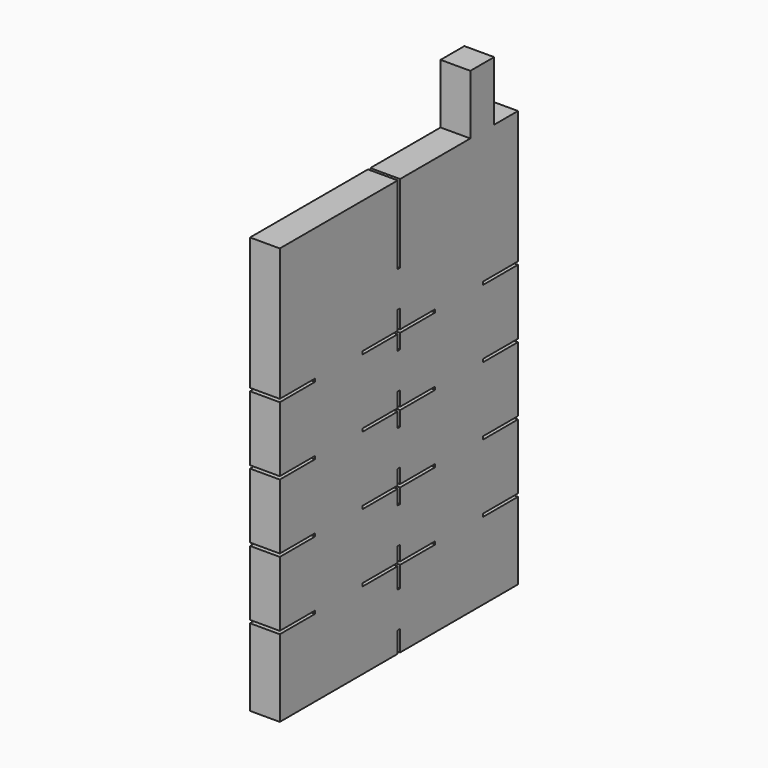
from build123d import *

# Parameters (mm, degrees)
F1_DEPTH = 5
F2_DEPTH = 10


# Not quite as in the source:
# - a feature names something its author has since deleted; it is built from what else it names


with BuildPart() as f1:
    # F0 (on Right) → F1 (new body)
    with BuildSketch(Plane.YZ):
        Polygon((11.5, 0), (0, 0), (0, -12.238), (7.3750000447, -12.238), (7.3750000447, -12.738), (0, -12.738), (0, -23.672), (7.3750000447, -23.672), (7.3750000447, -24.172), (0, -24.172), (0, -35.106), (7.3750000447, -35.106), (7.3750000447, -35.606), (0, -35.606), (0, -46.54), (7.3750000447, -46.54), (7.3750000447, -47.04), (0, -47.04), (0, -60), (24.75, -60), (24.75, -56.52), (25.25, -56.52), (25.25, -60), (50, -60), (50, -47.04), (42.6249988377, -47.04), (42.6249988377, -46.54), (50, -46.54), (50, -35.606), (42.6249988377, -35.606), (42.6249988377, -35.106), (50, -35.106), (50, -24.172), (42.6249988377, -24.172), (42.6249988377, -23.672), (50, -23.672), (50, -12.738), (42.6249988377, -12.738), (42.6249988377, -12.238), (50, -12.238), (50, 0), (45, 0), (45, 15), (45, 19.999999553), (40, 19.999999553), (40, 15), (40, 0), (37.625, 0), (35.125, 0), (25.25, 0), (25.25, -1.304), (25.25, -3.119), (24.75, -3.119), (24.75, 0), (14.875, 0), (12.375, 0), align=None)
        Polygon((25.25, -44.073), (25.25, -46.54), (32.625, -46.54), (32.625, -47.04), (25.25, -47.04), (25.25, -50.52), (24.75, -50.52), (24.75, -47.04), (17.375, -47.04), (17.375, -46.54), (24.75, -46.54), (24.75, -44.073), align=None, mode=Mode.SUBTRACT)
        Polygon((25.25, -32.639), (25.25, -35.106), (32.625, -35.106), (32.625, -35.606), (25.25, -35.606), (25.25, -38.073), (24.75, -38.073), (24.75, -35.606), (17.375, -35.606), (17.375, -35.106), (24.75, -35.106), (24.75, -32.639), align=None, mode=Mode.SUBTRACT)
        Polygon((25.25, -21.205), (25.25, -23.672), (32.625, -23.672), (32.625, -24.172), (25.25, -24.172), (25.25, -26.639), (24.75, -26.639), (24.75, -24.172), (17.375, -24.172), (17.375, -23.672), (24.75, -23.672), (24.75, -21.205), align=None, mode=Mode.SUBTRACT)
        Polygon((25.25, -9.119), (25.25, -12.238), (32.625, -12.238), (32.625, -12.738), (25.25, -12.738), (25.25, -15.205), (24.75, -15.205), (24.75, -12.738), (17.375, -12.738), (17.375, -12.238), (24.75, -12.238), (24.75, -9.119), align=None, mode=Mode.SUBTRACT)
    extrude(amount=F1_DEPTH)

    # F2 (add): faces of the model
    f2_faces = [f1.faces().sort_by_distance(p)[0] for p in [
        (2.5, 32.625, 0),
        (2.5, 12.375, 0),
        (2.5, 47.5, 0),
    ]]
    extrude(f2_faces, amount=F2_DEPTH)


solid = f1.part
